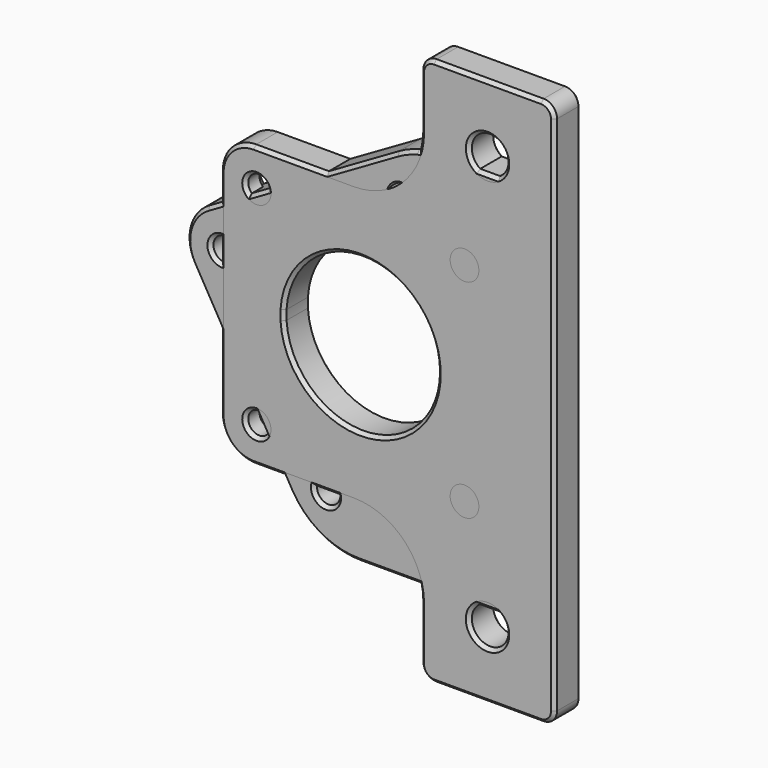
from build123d import *

# Parameters (mm, degrees)
F0_R           = 1.75
F0_R_2         = 12
F0_R_3         = 2.75
F1_DEPTH       = 5
F2_R           = 5
F3_SIZE        = 0.5
F4_R           = 11.5
F5_DEPTH       = 5
F6_D           = 5.5
F6_DEPTH       = 17
F6_TIP         = 1.6523667023
F7_D           = 3.3
F7_DEPTH       = 17
F7_CBORE_D     = 6.5
F7_CBORE_DEPTH = 2.4
F7_TIP         = 0.9914200214
F8_R           = 10
F9_R           = 5
F10_R          = 2
F11_SIZE       = 0.5


with BuildPart() as f1:
    # F0 (on Front) → F1 (new body)
    with BuildSketch(Plane.XZ):
        with BuildLine():
            Line((20, -7.3634480157), (-0.5940647845, 28.3065185255))
            ThreePointArc((-0.5940647845, 28.3065185255), (-2.137762574, 27.7946947913), (-3.5980762114, 27.0788383249))
            Line((-3.5980762114, 27.0788383249), (-31.9903810568, 10.6865334795))
            ThreePointArc((-31.9903810568, 10.6865334795), (-34.7859360145, 7.0432953274), (-34.1865334795, 2.4903810568))
            Line((-34.1865334795, 2.4903810568), (-19.6506350946, -22.6865334795))
            ThreePointArc((-19.6506350946, -22.6865334795), (-17.3449783133, -25.5525429024), (-14.2795100083, -27.585512965))
            Line((-14.2795100083, -27.585512965), (20, -7.7942286341))
            Line((20, -7.7942286341), (20, -7.3634480157))
        make_face()
        with Locations((-14.1715636316, -21.1665636316)):
            Circle(F0_R, mode=Mode.SUBTRACT)
        with Locations((12.6665636316, -5.6715636316)):
            Circle(F0_R, mode=Mode.SUBTRACT)
        with Locations((-29.6665636316, 5.6715636316)):
            Circle(F0_R, mode=Mode.SUBTRACT)
        with Locations((-8.5, 0)):
            Circle(F0_R_2, mode=Mode.SUBTRACT)
        with Locations((-2.8284363684, 21.1665636316)):
            Circle(F0_R, mode=Mode.SUBTRACT)
        with BuildLine():
            ThreePointArc((2.4019237886, 28.6865334795), (0.8919271913, 28.5911506626), (-0.5940647845, 28.3065185255))
            Line((-0.5940647845, 28.3065185255), (20, -7.3634480157))
            Line((20, -7.3634480157), (20, 28.6865334795))
            Line((20, 28.6865334795), (2.4019237886, 28.6865334795))
        make_face()
        with Locations((10, 20)):
            Circle(F0_R_3, mode=Mode.SUBTRACT)
        with BuildLine():
            Line((20, -28.6865334795), (20, -7.7942286341))
            Line((20, -7.7942286341), (-14.2795100083, -27.585512965))
            ThreePointArc((-14.2795100083, -27.585512965), (-11.8285681928, -28.408046902), (-9.2583302492, -28.6865334795))
            Line((-9.2583302492, -28.6865334795), (20, -28.6865334795))
        make_face()
        with Locations((10, -20)):
            Circle(F0_R_3, mode=Mode.SUBTRACT)
    extrude(amount=F1_DEPTH)

    # F2
    f2_edges = [f1.edges().sort_by_distance(p)[0] for p in [
        (20, -2.5, -28.686533),
        (20, -2.5, 28.686533),
    ]]
    fillet(f2_edges, radius=F2_R)

    # F3
    f3_edges = [f1.edges().sort_by_distance(p)[0] for p in [
        (8.700962, -5, 28.686533),
        (18.535534, -5, 27.222067),
        (-0.703905, -5, 28.277643),
        (20, -5, 0),
        (-17.794229, -5, 18.882686),
        (18.535534, -5, -27.222067),
        (-34.785936, -5, 7.043295),
        (2.870835, -5, -28.686533),
        (-26.918584, -5, -10.098076),
        (-15.25833, -5, -27.078838),
        (-15.921564, -5, -21.166564),
        (10.916564, -5, -5.671564),
        (-31.416564, -5, 5.671564),
        (-20.5, -5, 0),
        (-4.578436, -5, 21.166564),
        (7.25, -5, 20),
        (7.25, -5, -20),
        (8.700962, 0, 28.686533),
        (18.535534, 0, 27.222067),
        (-0.703905, 0, 28.277643),
        (20, 0, 0),
        (-17.794229, 0, 18.882686),
        (18.535534, 0, -27.222067),
        (-34.785936, 0, 7.043295),
        (2.870835, 0, -28.686533),
        (-26.918584, 0, -10.098076),
        (-15.25833, 0, -27.078838),
        (-15.921564, 0, -21.166564),
        (10.916564, 0, -5.671564),
        (-31.416564, 0, 5.671564),
        (-20.5, 0, 0),
        (-4.578436, 0, 21.166564),
        (7.25, 0, 20),
        (7.25, 0, -20),
    ]]
    chamfer(f3_edges, length=F3_SIZE)


with BuildPart() as f5:
    # F4 (on Front) → F5 (new body)
    with BuildSketch(Plane.XZ):
        Polygon((0, 41), (0, 21), (-30, 21), (-30, -21), (0, -21), (0, -41), (20, -41), (20, 41), align=None)
        with Locations((-9, 0)):
            Circle(F4_R, mode=Mode.SUBTRACT)
    extrude(amount=F5_DEPTH)

    # F6
    with Locations(Plane(origin=(0, 0, 0), x_dir=(1, 0, 0), z_dir=(0, 1, 0))):
        with Locations((10, -31), (10, 31)):
            Hole(F6_D / 2, depth=F6_DEPTH)
            with Locations((0, 0, -(F6_DEPTH + F6_TIP / 2))):  # 118° drill point
                Cone(0, F6_D / 2, F6_TIP, mode=Mode.SUBTRACT)

    # F7
    with Locations(Plane(origin=(0, 0, 0), x_dir=(1, 0, 0), z_dir=(0, 1, 0))):
        with Locations((-24.5563491861, -15.5563491861), (-24.5563491861, 15.5563491861), (6.5563491861, 15.5563491861), (6.5563491861, -15.5563491861)):
            CounterBoreHole(F7_D / 2, F7_CBORE_D / 2, F7_CBORE_DEPTH, depth=F7_DEPTH)
            with Locations((0, 0, -(F7_DEPTH + F7_TIP / 2))):  # 118° drill point
                Cone(0, F7_D / 2, F7_TIP, mode=Mode.SUBTRACT)

    # F8
    f8_edges = [f5.edges().sort_by_distance(p)[0] for p in [
        (0, -2.5, -21),
        (0, -2.5, 21),
    ]]
    fillet(f8_edges, radius=F8_R)

    # F9
    f9_edges = [f5.edges().sort_by_distance(p)[0] for p in [
        (-30, -2.5, 21),
        (-30, -2.5, -21),
    ]]
    fillet(f9_edges, radius=F9_R)

    # F10
    f10_edges = [f5.edges().sort_by_distance(p)[0] for p in [
        (20, -2.5, 41),
        (20, -2.5, -41),
        (0, -2.5, 41),
        (0, -2.5, -41),
    ]]
    fillet(f10_edges, radius=F10_R)

    # F11
    f11_edges = [f5.edges().sort_by_distance(p)[0] for p in [
        (0, -5, 35),
        (0.585786, -5, 40.414214),
        (-2.928932, -5, 23.928932),
        (10, -5, 41),
        (-17.5, -5, 21),
        (19.414214, -5, 40.414214),
        (-28.535534, -5, 19.535534),
        (20, -5, 0),
        (-30, -5, 0),
        (19.414214, -5, -40.414214),
        (-28.535534, -5, -19.535534),
        (10, -5, -41),
        (-17.5, -5, -21),
        (0.585786, -5, -40.414214),
        (-2.928932, -5, -23.928932),
        (0, -5, -35),
        (-26.206349, -5, -15.556349),
        (7.25, -5, -31),
        (4.906349, -5, -15.556349),
        (-26.206349, -5, 15.556349),
        (-20.5, -5, 0),
        (4.906349, -5, 15.556349),
        (7.25, -5, 31),
        (0, 0, 35),
        (0.585786, 0, 40.414214),
        (-2.928932, 0, 23.928932),
        (10, 0, 41),
        (-17.5, 0, 21),
        (19.414214, 0, 40.414214),
        (-28.535534, 0, 19.535534),
        (20, 0, 0),
        (-30, 0, 0),
        (19.414214, 0, -40.414214),
        (-28.535534, 0, -19.535534),
        (10, 0, -41),
        (-17.5, 0, -21),
        (0.585786, 0, -40.414214),
        (-2.928932, 0, -23.928932),
        (0, 0, -35),
        (-27.806349, 0, -15.556349),
        (7.25, 0, -31),
        (3.306349, 0, -15.556349),
        (-27.806349, 0, 15.556349),
        (-20.5, 0, 0),
        (3.306349, 0, 15.556349),
        (7.25, 0, 31),
    ]]
    chamfer(f11_edges, length=F11_SIZE)


solid = Compound([f1.part, f5.part])
